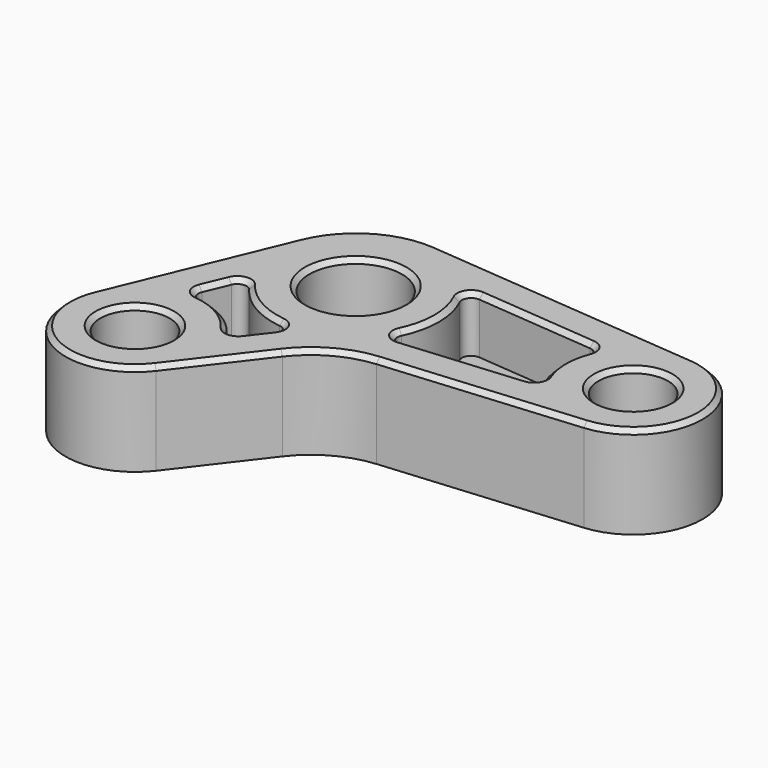
from build123d import *

# Parameters (mm, degrees)
F0_R     = 7.5
F0_R_2   = 10
F1_DEPTH = 20
F2_R     = 20
F3_T     = -8
F4_R     = 2
F6_SIZE  = 1


# Not quite as in the source:
# - two fillets or chamfers of one size are made in one step


with BuildPart() as f1:
    # F0 (on Top) → F1 (new body)
    with BuildSketch(Plane.XY):
        with BuildLine():
            Line((-18.6164580262, 7.8960385923), (-33.8581929877, -28.9007646659))
            ThreePointArc((-33.8581929877, -28.9007646659), (-27.5, -47.6313972081), (-8.0996998956, -43.7724375865))
            Line((-8.0996998956, -43.7724375865), (10.6191461494, -19.3775624703))
            Line((10.6191461494, -19.3775624703), (61.3073361412, -14.9429204714))
            ThreePointArc((61.3073361412, -14.9429204714), (75, 0), (61.3073361412, 14.9429204714))
            Line((61.3073361412, 14.9429204714), (1.604247479, 20.1662639068))
            ThreePointArc((1.604247479, 20.1662639068), (-10.5143325391, 17.3406073584), (-18.6164580262, 7.8960385923))
        make_face()
        with Locations((-20, -34.6410161514)):
            Circle(F0_R, mode=Mode.SUBTRACT)
        Circle(F0_R_2, mode=Mode.SUBTRACT)
        with Locations((60, 0)):
            Circle(F0_R, mode=Mode.SUBTRACT)
    extrude(amount=F1_DEPTH)

    # F2
    f2_edges = [f1.edges().sort_by_distance(p)[0] for p in [
        (10.619146, -19.377562, 10),
    ]]
    fillet(f2_edges, radius=F2_R)

    # F3
    f3_openings = [f1.faces().sort_by_distance(p)[0] for p in [
        (14.636401, -7.453279, 20),
    ]]
    offset(amount=F3_T, openings=f3_openings)

    # F4
    f4_edges = [f1.edges().sort_by_distance(p)[0] for p in [
        (-6.027772, -27.930812, 14),
        (13.849674, -11.497241, 14),
        (2.246879, -17.859214, 14),
        (46.833398, -8.178667, 14),
        (-21.174906, -19.185609, 14),
        (-16.348079, -7.532617, 14),
        (14.22329, 11.031682, 14),
        (46.833398, 8.178667, 14),
    ]]
    fillet(f4_edges, radius=F4_R)

    # F6
    f6_edges = [f1.edges().sort_by_distance(p)[0] for p in [
        (40.346603, -16.776747, 20),
        (-10, 0, 20),
        (31.29601, -9.538013, 20),
        (31.044956, 9.559977, 20),
        (17.546547, -4.014808, 20),
        (17.547047, 4.012624, 20),
        (-8.997951, -15.58964, 20),
        (44.5, 0, 20),
        (-27.5, -34.641016, 20),
        (-12.25, -21.217622, 20),
        (-2.661098, -23.543277, 20),
        (-18.959422, -13.836957, 20),
        (52.5, 0, 20),
        (18.453201, -10.662615, 20),
        (16.373656, -9.84693, 20),
        (45.430722, -7.49354, 20),
        (16.366311, 9.828794, 20),
        (45.430722, 7.49354, 20),
        (-1.418891, -35.065838, 20),
        (11.509209, -20.999932, 20),
        (75, 0, 20),
        (31.455792, 17.554592, 20),
        (-10.514333, 17.340607, 20),
        (-26.237326, -10.502363, 20),
        (-27.5, -47.631397, 20),
        (-0.936161, -21.297027, 20),
        (-0.501696, -19.09992, 20),
        (-5.851945, -26.379688, 20),
        (-16.270071, -9.986458, 20),
        (-19.919507, -18.257777, 20),
    ]]
    chamfer(f6_edges, length=F6_SIZE)


solid = f1.part
